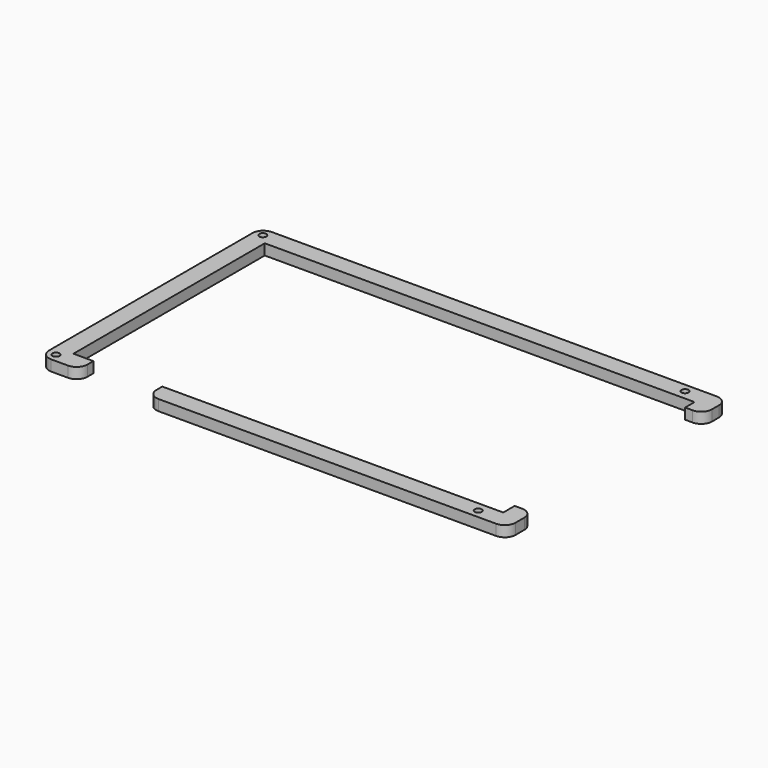
from build123d import *

# Parameters (mm, degrees)
F1_DEPTH = 5
F2_D     = 3.3
F2_2_D   = 3.3
F3_R     = 5
F3_2_R   = 5


# Not quite as in the source:
# - two fillets or chamfers of one size are made in one step


with BuildPart() as f1:
    # F0 (on Top) → F1 (new body)
    with BuildSketch(Plane.XY):
        Polygon((115.4999993443, 64.5), (103, 64.5), (-57.083491236, 64.5), (-83.2366272807, 64.5), (-101, 64.5), (-101, -63.5), (-83.2366272807, -63.5), (-83.2366272807, -55), (-92.5, -55), (-92.5, 56), (-83.0929607174, 56), (-57.083491236, 56), (103, 56), (106.9999993443, 56), (106.9999993443, 50.5), (115.4999993443, 50.5), align=None)
    extrude(amount=F1_DEPTH)

    # F2 (through all)
    with Locations(Plane(origin=(0, 0, 0), x_dir=(1, 0, 0), z_dir=(0, 0, -1))):
        with Locations((-97, -60.5), (99, -60.5), (-97, 59.5), (99, 59.5)):
            Hole(F2_D / 2)

    # F3
    f3_edges = [f1.edges().sort_by_distance(p)[0] for p in [
        (-101, 64.5, 2.5),
        (115.499999, 64.5, 2.5),
        (-101, -63.5, 2.5),
        (-83.236627, -63.5, 2.5),
        (115.499999, 50.5, 2.5),
    ]]
    fillet(f3_edges, radius=F3_R)


with BuildPart() as f1b:
    # F0 (on Top) → F1, piece 2 (new body)
    with BuildSketch(Plane.XY):
        Polygon((-51.2366272807, -63.5), (103, -63.5), (115.4999993443, -63.5), (115.4999993443, -48.3833029866), (106.9999993443, -48.3833029866), (106.9999993443, -55), (103, -55), (-51.2366272807, -55), align=None)
    extrude(amount=F1_DEPTH)

    # F2#2 (through all)
    with Locations(Plane(origin=(0, 0, 0), x_dir=(1, 0, 0), z_dir=(0, 0, -1))):
        with Locations((-97, -60.5), (99, -60.5), (-97, 59.5), (99, 59.5)):
            Hole(F2_2_D / 2)

    # F3#2
    f3_2_edges = [f1b.edges().sort_by_distance(p)[0] for p in [
        (-51.236627, -63.5, 2.5),
        (115.499999, -63.5, 2.5),
        (115.499999, -48.383303, 2.5),
    ]]
    fillet(f3_2_edges, radius=F3_2_R)


solid = Compound([f1.part, f1b.part])
